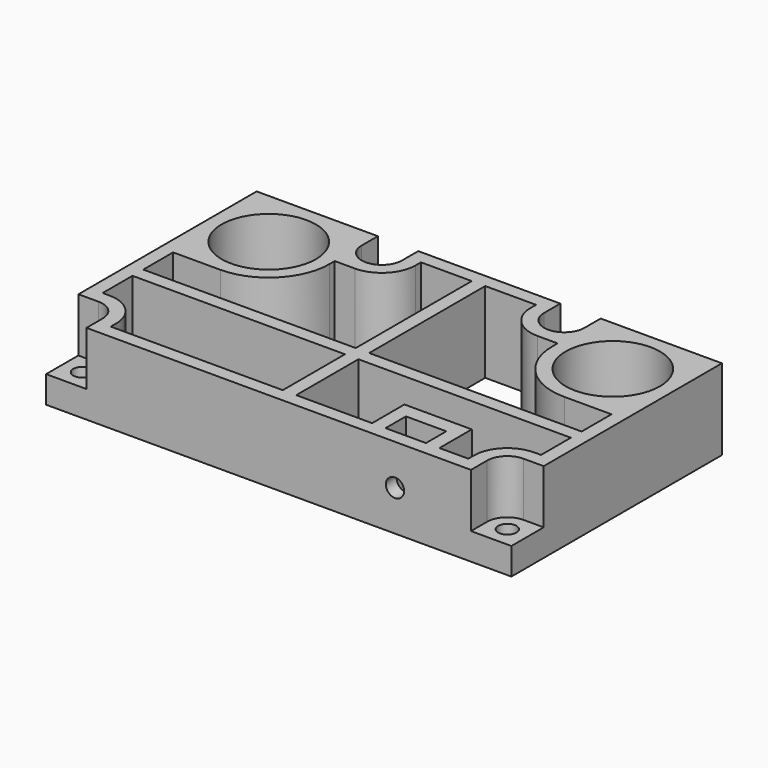
from build123d import *

# Parameters (mm, degrees)
F0_W      = 109.6809846
F0_H      = 62.036204
F0_R      = 2.15265
F0_W_2    = 9.525
F0_H_2    = 6
F0_R_2    = 11.1125
F1_DEPTH  = 19.05
F2_W      = 9.525
F2_H      = 9.525
F3_DEPTH  = 12.7
F4_R      = 4.76249
F6_DEPTH  = 19.05
F7_R      = 2.15265
F8_DEPTH  = 3.175
F9_R      = 1.7272
F10_DEPTH = 3.525


# Not quite as in the source:
# - a fillet or chamfer is up to 0.001 mm smaller than in the source, because OpenCascade refuses the exact size


with BuildPart() as f1:
    # F0 (on Top) → F1 (new body)
    with BuildSketch(Plane.XY):
        with Locations((0, -16.730602)):
            Rectangle(F0_W, F0_H)
        with Locations((-50.0779923, -42.986204)):
            Circle(F0_R, mode=Mode.SUBTRACT)
        with Locations((27.406219, -41.573704)):
            Rectangle(F0_W_2, F0_H_2, mode=Mode.SUBTRACT)
        with Locations((50.0779923, -42.986204)):
            Circle(F0_R, mode=Mode.SUBTRACT)
        with Locations((-40.5529923, 0)):
            Circle(F0_R_2, mode=Mode.SUBTRACT)
        with Locations((-21.5029923, 9.525)):
            Circle(F0_R, mode=Mode.SUBTRACT)
        with Locations((21.5029923, 9.525)):
            Circle(F0_R, mode=Mode.SUBTRACT)
        with Locations((40.5529923, 0)):
            Circle(F0_R_2, mode=Mode.SUBTRACT)
    extrude(amount=F1_DEPTH)

    # F2 (on face) → F3 (cut)
    with BuildSketch(Plane.XY.offset(19.05)):
        with Locations((-21.5029923, 9.525)):
            Rectangle(F2_W, F2_H)
        with Locations((21.5029923, 9.525)):
            Rectangle(F2_W, F2_H)
        with Locations((50.0779923, -42.986204)):
            Rectangle(F2_W, F2_H)
        with Locations((-50.0779923, -42.986204)):
            Rectangle(F2_W, F2_H)
    extrude(amount=-F3_DEPTH, mode=Mode.SUBTRACT)

    # F4 (radius 4.7625 in the source; OpenCascade refuses exactly that, so slightly less here)
    f4_edges = [f1.edges().sort_by_distance(p)[0] for p in [
        (-45.315492, -38.223704, 12.7),
        (45.315492, -38.223704, 12.7),
        (16.740492, 4.7625, 12.7),
        (26.265492, 4.7625, 12.7),
        (-16.740492, 4.7625, 12.7),
        (-26.265492, 4.7625, 12.7),
    ]]
    fillet(f4_edges, radius=F4_R)

    # F5 (on face) → F6 (cut, through all)
    with BuildSketch(Plane.XY.offset(19.05)):
        with BuildLine():
            Line((-51.6654923, -23.080602), (-1.5875, -23.080602))
            Line((-1.5875, -23.080602), (-1.5875, 11.1125))
            Line((-1.5875, 11.1125), (-13.5654923, 11.1125))
            Line((-13.5654923, 11.1125), (-13.5654923, 9.525))
            ThreePointArc((-13.5654923, 9.525), (-15.8903322243, 3.9123399243), (-21.5029923, 1.5875))
            Line((-21.5029923, 1.5875), (-26.2654923, 1.5875))
            Line((-26.2654923, 1.5875), (-26.2654923, 0))
            ThreePointArc((-26.2654923, 0), (-30.4502041638, -10.1027881362), (-40.5529923, -14.2875))
            Line((-40.5529923, -14.2875), (-51.6654923, -14.2875))
            Line((-51.6654923, -14.2875), (-51.6654923, -23.080602))
        make_face()
        with BuildLine():
            Line((-1.5875, -44.573704), (-1.5875, -26.255602))
            Line((-1.5875, -26.255602), (-51.6654923, -26.255602))
            Line((-51.6654923, -26.255602), (-51.6654923, -35.048704))
            Line((-51.6654923, -35.048704), (-50.0779923, -35.048704))
            ThreePointArc((-50.0779923, -35.048704), (-44.4653322243, -37.3735439243), (-42.1404923, -42.986204))
            Line((-42.1404923, -42.986204), (-42.1404923, -44.573704))
            Line((-42.1404923, -44.573704), (-1.5875, -44.573704))
        make_face()
        with BuildLine():
            Line((1.5875, -23.080602), (51.6654923, -23.080602))
            Line((51.6654923, -23.080602), (51.6654923, -14.2875))
            Line((51.6654923, -14.2875), (40.5529923, -14.2875))
            ThreePointArc((40.5529923, -14.2875), (30.4502041638, -10.1027881362), (26.2654923, 0))
            Line((26.2654923, 0), (26.2654923, 1.5875))
            Line((26.2654923, 1.5875), (21.5029923, 1.5875))
            ThreePointArc((21.5029923, 1.5875), (15.8903322243, 3.9123399243), (13.5654923, 9.525))
            Line((13.5654923, 9.525), (13.5654923, 11.1125))
            Line((13.5654923, 11.1125), (1.5875, 11.1125))
            Line((1.5875, 11.1125), (1.5875, -23.080602))
        make_face()
        with BuildLine():
            Line((51.6654923, -26.255602), (1.5875, -26.255602))
            Line((1.5875, -26.255602), (1.5875, -44.573704))
            Line((1.5875, -44.573704), (19.468719, -44.573704))
            Line((19.468719, -44.573704), (19.468719, -35.048704))
            Line((19.468719, -35.048704), (35.343719, -35.048704))
            Line((35.343719, -35.048704), (35.343719, -44.573704))
            Line((35.343719, -44.573704), (42.1404923, -44.573704))
            Line((42.1404923, -44.573704), (42.1404923, -42.986204))
            ThreePointArc((42.1404923, -42.986204), (44.4653322243, -37.3735439243), (50.0779923, -35.048704))
            Line((50.0779923, -35.048704), (51.6654923, -35.048704))
            Line((51.6654923, -35.048704), (51.6654923, -26.255602))
        make_face()
    extrude(amount=-F6_DEPTH, mode=Mode.SUBTRACT)

    # F7 (on face) → F8 (cut, through all)
    with BuildSketch(Plane.XZ.offset(47.748704)):
        with Locations((27.406219, 9.525)):
            Circle(F7_R)
    extrude(amount=-F8_DEPTH, mode=Mode.SUBTRACT)

    # F9 (on face) → F10 (cut, through all)
    with BuildSketch(Plane.XZ.offset(38.573704)):
        with Locations((27.406219, 9.525)):
            Circle(F9_R)
    extrude(amount=-F10_DEPTH, mode=Mode.SUBTRACT)


solid = f1.part
